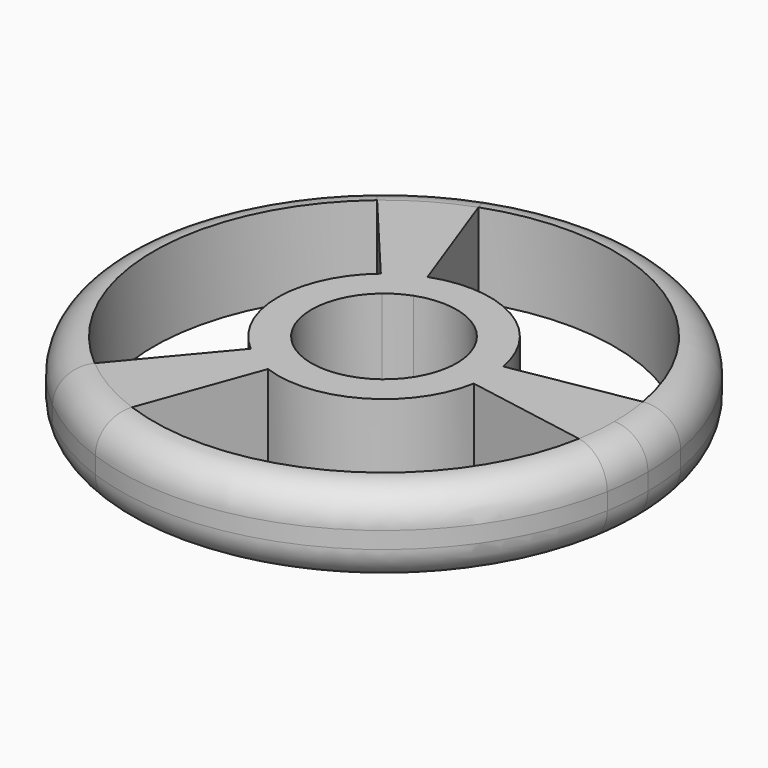
from build123d import *

# Parameters (mm, degrees)
F1_DEPTH = 12.7
F2_R     = 5.07999


# Not quite as in the source:
# - a fillet or chamfer is up to 0.001 mm smaller than in the source, because OpenCascade refuses the exact size


with BuildPart() as f1:
    # F0 (on Top) → F1 (new body)
    with BuildSketch(Plane.XY):
        with BuildLine():
            ThreePointArc((-27.1257893014, 52.8568671478), (-22.1396459711, 56.3482022942), (-16.6229893761, 58.9206615119))
            Line((-16.6229893761, 58.9206615119), (-18.3604517042, 63.6943000255))
            ThreePointArc((-18.3604517042, 63.6943000255), (-24.6796459711, 60.7476113455), (-30.3911503586, 56.7483729188))
            Line((-30.3911503586, 56.7483729188), (-27.1257893014, 52.8568671478))
        make_face()
        with BuildLine():
            ThreePointArc((-27.1257893014, -0.6436767596), (-39.5996459711, 26.1065951941), (-27.1257893014, 52.8568671478))
            Line((-27.1257893014, 52.8568671478), (-30.3911503586, 56.7483729188))
            ThreePointArc((-30.3911503586, 56.7483729188), (-44.6796459711, 26.1065951941), (-30.3911503586, -4.5351825307))
            Line((-30.3911503586, -4.5351825307), (-27.1257893014, -0.6436767596))
        make_face()
        with BuildLine():
            Line((-18.3604517042, -11.4811096374), (-16.6229893761, -6.7074711238))
            ThreePointArc((-16.6229893761, -6.7074711238), (-22.1396459711, -4.1350119061), (-27.1257893014, -0.6436767596))
            Line((-27.1257893014, -0.6436767596), (-30.3911503586, -4.5351825307))
            ThreePointArc((-30.3911503586, -4.5351825307), (-24.6796459711, -8.5344209573), (-18.3604517042, -11.4811096374))
        make_face()
        with BuildLine():
            Line((34.7126641494, 19.1606680874), (29.709840764, 20.04280083))
            ThreePointArc((29.709840764, 20.04280083), (12.7803540289, -4.1350119061), (-16.6229893761, -6.7074711238))
            Line((-16.6229893761, -6.7074711238), (-18.3604517042, -11.4811096374))
            ThreePointArc((-18.3604517042, -11.4811096374), (15.3203540289, -8.5344209573), (34.7126641494, 19.1606680874))
        make_face()
        with BuildLine():
            Line((34.7126641494, 33.0525223008), (29.709840764, 32.1703895582))
            ThreePointArc((29.709840764, 32.1703895582), (30.1074728862, 29.1500737308), (30.2403540289, 26.1065951941))
            ThreePointArc((30.2403540289, 26.1065951941), (30.1074728862, 23.0631166573), (29.709840764, 20.04280083))
            Line((29.709840764, 20.04280083), (34.7126641494, 19.1606680874))
            ThreePointArc((34.7126641494, 19.1606680874), (35.1681419525, 22.6203654842), (35.3203540289, 26.1065951941))
            ThreePointArc((35.3203540289, 26.1065951941), (35.1681419525, 29.592824904), (34.7126641494, 33.0525223008))
        make_face()
        with BuildLine():
            ThreePointArc((-15.0156707349, 38.4245898394), (-12.7196459711, 40.0322836869), (-10.1793298758, 41.2168525363))
            Line((-10.1793298758, 41.2168525363), (-16.6229893761, 58.9206615119))
            ThreePointArc((-16.6229893761, 58.9206615119), (-22.1396459711, 56.3482022942), (-27.1257893014, 52.8568671478))
            Line((-27.1257893014, 52.8568671478), (-15.0156707349, 38.4245898394))
        make_face()
        with BuildLine():
            ThreePointArc((-8.4418675477, 36.4432140227), (0.8203540289, 35.6328746357), (6.153239312, 28.0167251484))
            Line((6.153239312, 28.0167251484), (11.1560626973, 28.898857891))
            ThreePointArc((11.1560626973, 28.898857891), (3.3603540289, 40.0322836869), (-10.1793298758, 41.2168525363))
            Line((-10.1793298758, 41.2168525363), (-8.4418675477, 36.4432140227))
        make_face()
        with BuildLine():
            ThreePointArc((-11.7503096777, 17.6801063198), (-15.6796459711, 26.1065951941), (-11.7503096777, 34.5330840684))
            Line((-11.7503096777, 34.5330840684), (-15.0156707349, 38.4245898394))
            ThreePointArc((-15.0156707349, 38.4245898394), (-20.7596459711, 26.1065951941), (-15.0156707349, 13.7886005487))
            Line((-15.0156707349, 13.7886005487), (-11.7503096777, 17.6801063198))
        make_face()
        with BuildLine():
            ThreePointArc((-11.7503096777, 34.5330840684), (-10.1796459711, 35.6328746357), (-8.4418675477, 36.4432140227))
            Line((-8.4418675477, 36.4432140227), (-10.1793298758, 41.2168525363))
            ThreePointArc((-10.1793298758, 41.2168525363), (-12.7196459711, 40.0322836869), (-15.0156707349, 38.4245898394))
            Line((-15.0156707349, 38.4245898394), (-11.7503096777, 34.5330840684))
        make_face()
        with BuildLine():
            Line((11.1560626973, 23.3143324972), (6.153239312, 24.1964652397))
            ThreePointArc((6.153239312, 24.1964652397), (0.8203540289, 16.5803157525), (-8.4418675477, 15.7699763654))
            Line((-8.4418675477, 15.7699763654), (-10.1793298758, 10.9963378518))
            ThreePointArc((-10.1793298758, 10.9963378518), (3.3603540289, 12.1809067012), (11.1560626973, 23.3143324972))
        make_face()
        with BuildLine():
            ThreePointArc((6.153239312, 28.0167251484), (6.2784957079, 27.0653083643), (6.3203540289, 26.1065951941))
            ThreePointArc((6.3203540289, 26.1065951941), (6.2784957079, 25.1478820239), (6.153239312, 24.1964652397))
            Line((6.153239312, 24.1964652397), (11.1560626973, 23.3143324972))
            ThreePointArc((11.1560626973, 23.3143324972), (11.3391647742, 24.7051308507), (11.4003540289, 26.1065951941))
            ThreePointArc((11.4003540289, 26.1065951941), (11.3391647742, 27.5080595375), (11.1560626973, 28.898857891))
            Line((11.1560626973, 28.898857891), (6.153239312, 28.0167251484))
        make_face()
        with BuildLine():
            Line((-10.1793298758, 10.9963378518), (-8.4418675477, 15.7699763654))
            ThreePointArc((-8.4418675477, 15.7699763654), (-10.1796459711, 16.5803157525), (-11.7503096777, 17.6801063198))
            Line((-11.7503096777, 17.6801063198), (-15.0156707349, 13.7886005487))
            ThreePointArc((-15.0156707349, 13.7886005487), (-12.7196459711, 12.1809067012), (-10.1793298758, 10.9963378518))
        make_face()
        with BuildLine():
            ThreePointArc((-16.6229893761, 58.9206615119), (12.7803540289, 56.3482022942), (29.709840764, 32.1703895582))
            Line((29.709840764, 32.1703895582), (34.7126641494, 33.0525223008))
            ThreePointArc((34.7126641494, 33.0525223008), (15.3203540289, 60.7476113455), (-18.3604517042, 63.6943000255))
            Line((-18.3604517042, 63.6943000255), (-16.6229893761, 58.9206615119))
        make_face()
        with BuildLine():
            Line((29.709840764, 32.1703895582), (11.1560626973, 28.898857891))
            ThreePointArc((11.1560626973, 28.898857891), (11.3391647742, 27.5080595375), (11.4003540289, 26.1065951941))
            ThreePointArc((11.4003540289, 26.1065951941), (11.3391647742, 24.7051308507), (11.1560626973, 23.3143324972))
            Line((11.1560626973, 23.3143324972), (29.709840764, 20.04280083))
            ThreePointArc((29.709840764, 20.04280083), (30.1074728862, 23.0631166573), (30.2403540289, 26.1065951941))
            ThreePointArc((30.2403540289, 26.1065951941), (30.1074728862, 29.1500737308), (29.709840764, 32.1703895582))
        make_face()
        with BuildLine():
            Line((-16.6229893761, -6.7074711238), (-10.1793298758, 10.9963378518))
            ThreePointArc((-10.1793298758, 10.9963378518), (-12.7196459711, 12.1809067012), (-15.0156707349, 13.7886005487))
            Line((-15.0156707349, 13.7886005487), (-27.1257893014, -0.6436767596))
            ThreePointArc((-27.1257893014, -0.6436767596), (-22.1396459711, -4.1350119061), (-16.6229893761, -6.7074711238))
        make_face()
    extrude(amount=F1_DEPTH)

    # F2 (radius 5.08 in the source; OpenCascade refuses exactly that, so slightly less here)
    f2_edges = [f1.edges().sort_by_distance(p)[0] for p in [
        (-44.071956, 19.160668, 12.7),
        (-44.071956, 19.160668, 0),
    ]]
    fillet(f2_edges, radius=F2_R)


solid = f1.part
